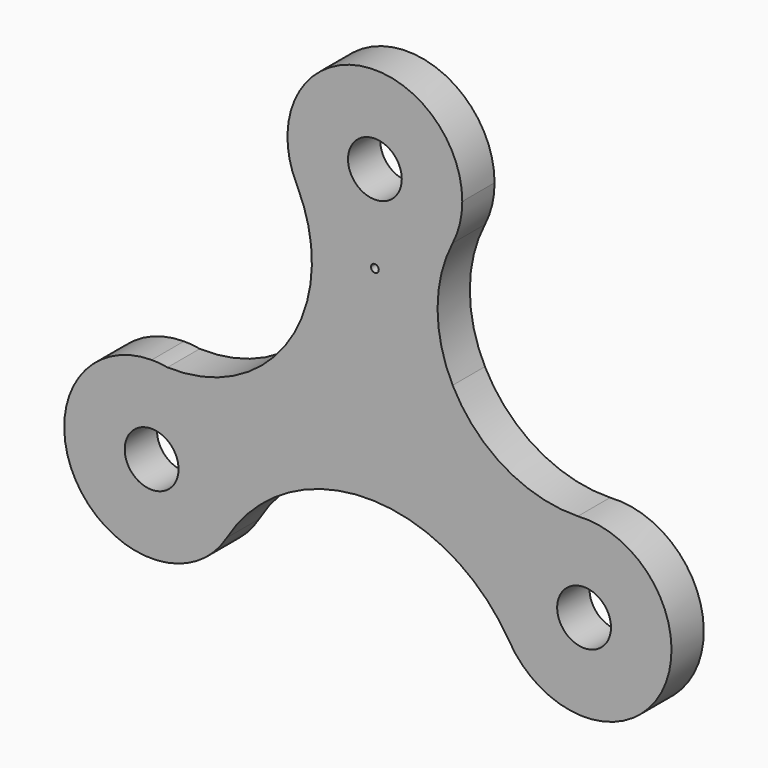
from build123d import *

# Parameters (mm, degrees)
F0_R     = 9.5
F0_R_2   = 4
F1_DEPTH = 6


with BuildPart() as f1:
    # F0 (on Front) → F1 (new body)
    with BuildSketch(Plane.XZ):
        with BuildLine():
            ThreePointArc((2.350153171, 12.7858038493), (1.1720328397, 12.8595060447), (0, 13))
            ThreePointArc((0, 13), (-11.2995091051, -6.4281485658), (11.1746035767, -6.6429086178))
            ThreePointArc((11.1746035767, -6.6429086178), (12.5353469536, -3.4445720709), (13, 0))
            ThreePointArc((13, 0), (9.9887935013, 8.320096417), (2.350153171, 12.7858038493))
        make_face()
        Circle(F0_R, mode=Mode.SUBTRACT)
        with BuildLine():
            ThreePointArc((2.350153171, 12.7858038493), (1.179947024, 12.9463402172), (0, 13))
            ThreePointArc((0, 13), (1.1720328397, 12.8595060447), (2.350153171, 12.7858038493))
        make_face()
        with BuildLine():
            ThreePointArc((13, 0), (12.5353469536, -3.4445720709), (11.1746035767, -6.6429086178))
            ThreePointArc((11.1746035767, -6.6429086178), (20.3927051131, 2.2823011589), (32.8593572911, 5.3179804839))
            ThreePointArc((32.8593572911, 5.3179804839), (22.0397803989, 11.649441895), (21.5996059124, 24.1776857522))
            ThreePointArc((21.5996059124, 24.1776857522), (13.63881463, 15.6701075209), (2.350153171, 12.7858038493))
            ThreePointArc((2.350153171, 12.7858038493), (9.9887935013, 8.320096417), (13, 0))
        make_face()
        with BuildLine():
            ThreePointArc((21.5996059124, 24.1776857522), (22.0397803989, 11.649441895), (32.8593572911, 5.3179804839))
            ThreePointArc((32.8593572911, 5.3179804839), (42.272310005, 9.0007955279), (46.2018025219, 18.3134693652))
            ThreePointArc((46.2018025219, 18.3134693652), (45.8389012751, 21.3636718342), (44.7704586601, 24.243578568))
            ThreePointArc((44.7704586601, 24.243578568), (33.1648335269, 31.3134167995), (21.5996059124, 24.1776857522))
        make_face()
        with BuildLine():
            ThreePointArc((46.2018025219, 18.3134693652), (42.272310005, 9.0007955279), (32.8593572911, 5.3179804839))
            ThreePointArc((32.8593572911, 5.3179804839), (44.5354086005, 1.9994233392), (53.1813680275, -6.5205755628))
            ThreePointArc((53.1813680275, -6.5205755628), (52.7786540902, 6.1760009355), (63.3931152108, 13.154428295))
            ThreePointArc((63.3931152108, 13.154428295), (52.487300782, 16.0212898755), (44.7704586601, 24.243578568))
            ThreePointArc((44.7704586601, 24.243578568), (45.8389012751, 21.3636718342), (46.2018025219, 18.3134693652))
        make_face()
        with BuildLine():
            ThreePointArc((21.5996059834, 42.9212888668), (23.8334826654, 33.549487301), (21.5996059124, 24.1776857522))
            ThreePointArc((21.5996059124, 24.1776857522), (33.1648335269, 31.3134167995), (44.7704586601, 24.243578568))
            ThreePointArc((44.7704586601, 24.243578568), (42.5243018444, 33.5494874141), (44.7704586914, 42.8553962526))
            ThreePointArc((44.7704586914, 42.8553962526), (40.2259887899, 37.846547159), (33.7803843902, 35.7983870449))
            ThreePointArc((33.7803843902, 35.7983870449), (33.7804919256, 35.7919466185), (33.7805277722, 35.7855053943))
            ThreePointArc((33.7805277722, 35.7855053943), (33.1953612977, 35.2068159906), (32.6232206536, 35.7983870449))
            ThreePointArc((32.6232206536, 35.7983870449), (26.1465368827, 37.8665664916), (21.5996059834, 42.9212888668))
        make_face()
        with BuildLine():
            ThreePointArc((63.3931152108, 13.154428295), (52.7786540902, 6.1760009355), (53.1813680275, -6.5205755628))
            ThreePointArc((53.1813680275, -6.5205755628), (67.7981541622, -12.3379567831), (77.3170911302, 0.1873056959))
            ThreePointArc((77.3170911302, 0.1873056959), (73.176783931, 9.7007616124), (63.3931152108, 13.154428295))
        make_face()
        with Locations((64.3170911302, 0.1873056959)):
            Circle(F0_R, mode=Mode.SUBTRACT)
        with BuildLine():
            ThreePointArc((46.2018025219, 48.7855053943), (30.1875492977, 61.4312271017), (21.5996059834, 42.9212888668))
            ThreePointArc((21.5996059834, 42.9212888668), (26.1465368827, 37.8665664916), (32.6232206536, 35.7983870449))
            ThreePointArc((32.6232206536, 35.7983870449), (33.2018025219, 36.3642306445), (33.7803843902, 35.7983870449))
            ThreePointArc((33.7803843902, 35.7983870449), (40.2259887899, 37.846547159), (44.7704586914, 42.8553962526))
            ThreePointArc((44.7704586914, 42.8553962526), (45.8389012832, 45.7353029587), (46.2018025219, 48.7855053943))
        make_face()
        with Locations((33.2018025219, 48.7855053943)):
            Circle(F0_R, mode=Mode.SUBTRACT)
        with Locations((33.2018025219, 48.7855053943)):
            Circle(F0_R)
        with Locations((33.2018025219, 48.7855053943)):
            Circle(F0_R_2, mode=Mode.SUBTRACT)
        Circle(F0_R)
        Circle(F0_R_2, mode=Mode.SUBTRACT)
        with Locations((64.3170911302, 0.1873056959)):
            Circle(F0_R)
        with Locations((64.3170911302, 0.1873056959)):
            Circle(F0_R_2, mode=Mode.SUBTRACT)
    extrude(amount=F1_DEPTH)


solid = f1.part
